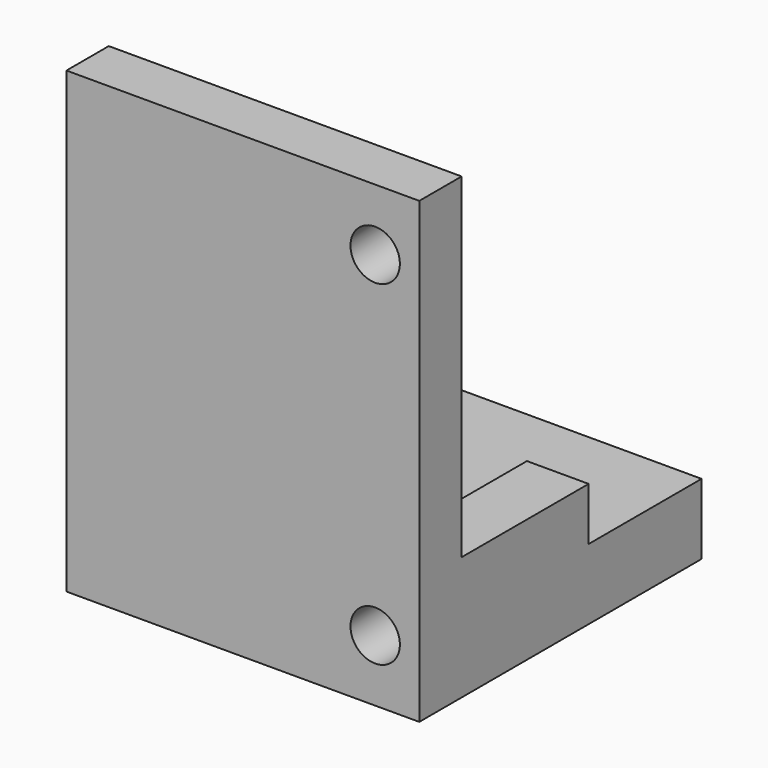
from build123d import *

# Parameters (mm, degrees)
F0_W      = 20
F0_H      = 20
F0_R      = 2.75
F1_DEPTH  = 4
F2_W      = 20
F2_H      = 26
F3_DEPTH  = 3
F5_W      = 5
F5_H      = 9
F6_DEPTH  = 3
F4_R      = 1.4
F7_DEPTH  = 10
F9_DEPTH  = 3
F10_SIZE2 = 1.49999
F10_SIZE  = 2.99999


# Not quite as in the source:
# - a fillet or chamfer is up to 0.001 mm smaller than in the source, because OpenCascade refuses the exact size


with BuildPart() as f1:
    # F0 (on Top) → F1 (new body)
    with BuildSketch(Plane.XY):
        with Locations((10, 10)):
            Rectangle(F0_W, F0_H)
        with Locations((10, 10)):
            Circle(F0_R, mode=Mode.SUBTRACT)
    extrude(amount=F1_DEPTH)

    # F2 (on face) → F3 (join)
    with BuildSketch(Plane.XZ):
        with Locations((10, 13)):
            Rectangle(F2_W, F2_H)
    extrude(amount=-F3_DEPTH)

    # F5 (on face) → F6 (join)
    with BuildSketch(Plane.XY.offset(4)):
        with Locations((17.5, 7.5)):
            Rectangle(F5_W, F5_H)
    extrude(amount=F6_DEPTH)

    # F4 (on face) → F7 (cut)
    with BuildSketch(Plane.XZ):
        with Locations((17.5, 3.5)):
            Circle(F4_R)
        with Locations((17.5, 22.5)):
            Circle(F4_R)
    extrude(amount=-F7_DEPTH, mode=Mode.SUBTRACT)

    # F8 (on face) → F9 (join)
    with BuildSketch(Plane(origin=(0, 0, 0), x_dir=(0, -1, 0), z_dir=(-1, 0, 0))):
        Polygon((-3, 4), (-3, 26), (-20, 4), align=None)
    extrude(amount=-F9_DEPTH)

    # F10 (size 3 and 1.5 in the source; OpenCascade refuses exactly that, so slightly less here)
    f10_edges = [f1.edges().sort_by_distance(p)[0] for p in [
        (15, 7.5, 7),
    ]]
    f10_side = f1.faces().sort_by_distance((15, 7.5, 5.5))[0]
    chamfer(f10_edges, length=F10_SIZE, length2=F10_SIZE2, reference=f10_side)


solid = f1.part
